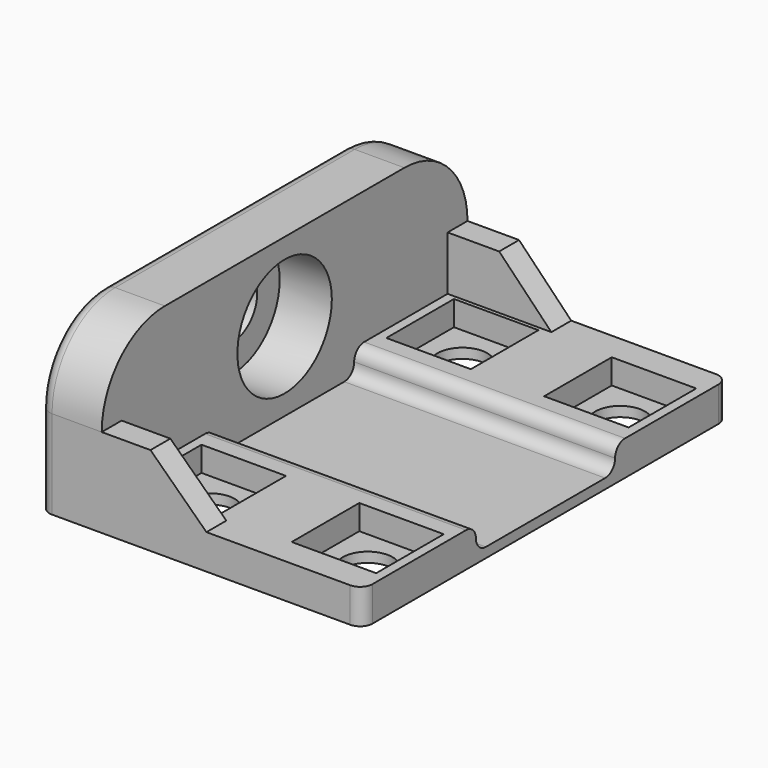
from build123d import *

# Parameters (mm, degrees)
F0_W           = 21
F0_H           = 36.8
F0_R           = 2
F1_DEPTH       = 0.8
F0_W_2         = 5
F2_DEPTH       = 13.5
F5_R           = 6.35
F6_D           = 5
F6_CBORE_D     = 9.5
F6_CBORE_DEPTH = 4.2
F7_W           = 10.5
F7_H           = 2
F7_R           = 2
F8_DEPTH       = 2
F9_DEPTH       = 6.35
F10_T4_DEPTH   = 35.8364431643
F10_T9_DEPTH   = 35.8364431643
F11_W          = 6.8
F11_H          = 6.8
F12_DEPTH      = 2
F13_R          = 0.99999


# Not quite as in the source:
# - a fillet or chamfer that OpenCascade refuses, or shapes differently, is made with other operations: its cross-section is extruded or revolved along the edge and cut away or added
# - a fillet or chamfer is up to 0.001 mm smaller than in the source, because OpenCascade refuses the exact size


with BuildPart() as f1:
    # F0 (on Top) → F1 (new body)
    with BuildSketch(Plane.XY):
        Rectangle(F0_W, F0_H)
        with Locations((-6.35, -12.7)):
            Circle(F0_R, mode=Mode.SUBTRACT)
        with Locations((6.35, -12.7)):
            Circle(F0_R, mode=Mode.SUBTRACT)
        with Locations((-6.35, 12.7)):
            Circle(F0_R, mode=Mode.SUBTRACT)
        with Locations((6.35, 12.7)):
            Circle(F0_R, mode=Mode.SUBTRACT)
    extrude(amount=F1_DEPTH)

    # F0 (on Top) → F2 (join)
    with BuildSketch(Plane.XY):
        with Locations((-13, 0)):
            Rectangle(F0_W_2, F0_H)
    extrude(amount=F2_DEPTH)

    # F5
    f5_edges = [f1.edges().sort_by_distance(p)[0] for p in [
        (-13, -18.4, 13.5),
        (-13, 18.4, 13.5),
    ]]
    fillet(f5_edges, radius=F5_R)

    # F6 (through all)
    with Locations(Plane.YZ.offset(-10.5)):
        with Locations((0, 7.15)):
            CounterBoreHole(F6_D / 2, F6_CBORE_D / 2, F6_CBORE_DEPTH)

    # F7 (on face) → F8 (join)
    with BuildSketch(Plane.XY.offset(0.8)):
        with Locations((-5.25, -17.4)):
            Rectangle(F7_W, F7_H)
        Polygon((-10.5, -16.4), (0, -16.4), (0, -18.4), (10.5, -18.4), (10.5, -7), (-10.5, -7), align=None)
        Polygon((-10.5, 16.4), (-10.5, 7), (10.5, 7), (10.5, 18.4), (0, 18.4), (0, 16.4), align=None)
        with Locations((-6.35, 12.7)):
            Circle(F7_R, mode=Mode.SUBTRACT)
        with Locations((6.35, 12.7)):
            Circle(F7_R, mode=Mode.SUBTRACT)
    extrude(amount=F8_DEPTH)

    # F7 (on face) → F9 (join)
    with BuildSketch(Plane.XY.offset(0.8)):
        with Locations((-5.25, -17.4)):
            Rectangle(F7_W, F7_H)
        with Locations((-5.25, 17.4)):
            Rectangle(F7_W, F7_H)
    extrude(amount=F9_DEPTH)

    # F10: chamfer of 6.35 x 6.5756174926 on 2 edges, made by hand


with BuildPart() as f10_tool2:
    # F10_s3 → F10_t4 (new body)
    with BuildSketch(Plane.XZ.offset(35.3182215821)):
        Polygon((-6.5756174926, 7.15), (0, 0.8), (0, 7.15), align=None)
    extrude(amount=-F10_T4_DEPTH)

    split(bisect_by=Plane.XY.offset(2.8), keep=Keep.TOP)


with BuildPart() as f1_1:
    add(f1.part)

    # F10_t1: cut F10_tool2
    add(f10_tool2.part, mode=Mode.SUBTRACT)


with BuildPart() as f10_tool7:
    # F10_s8 → F10_t9 (new body)
    with BuildSketch(Plane.XZ.offset(0.5182215821)):
        Polygon((-6.35, 7.15), (0, 0.5743825074), (0, 7.15), align=None)
    extrude(amount=-F10_T9_DEPTH)

    split(bisect_by=Plane.XY.offset(2.8), keep=Keep.TOP)


with BuildPart() as f1_2:
    add(f1_1.part)

    # F10_t6: cut F10_tool7
    add(f10_tool7.part, mode=Mode.SUBTRACT)

    # F11 (on face) → F12 (cut)
    with BuildSketch(Plane.XY.offset(2.8)):
        with Locations((-6.35, -12.7)):
            Rectangle(F11_W, F11_H)
        with Locations((6.35, -12.7)):
            Rectangle(F11_W, F11_H)
        with Locations((-6.35, 12.7)):
            Rectangle(F11_W, F11_H)
        with Locations((6.35, 12.7)):
            Rectangle(F11_W, F11_H)
    extrude(amount=-F12_DEPTH, mode=Mode.SUBTRACT)

    # F13 (radius 1 in the source; OpenCascade refuses exactly that, so slightly less here)
    f13_edges = [f1_2.edges().sort_by_distance(p)[0] for p in [
        (10.5, -18.4, 1.4),
        (10.5, 18.4, 1.4),
        (-15.5, -18.4, 3.575),
        (0, 7, 0.8),
        (0, -7, 0.8),
        (0, 7, 2.8),
        (0, -7, 2.8),
        (-15.5, 0, 13.5),
        (-15.5, -16.540128, 11.640128),
        (-15.5, 16.540128, 11.640128),
        (-15.5, 18.4, 3.575),
    ]]
    fillet(f13_edges, radius=F13_R)


solid = f1_2.part
